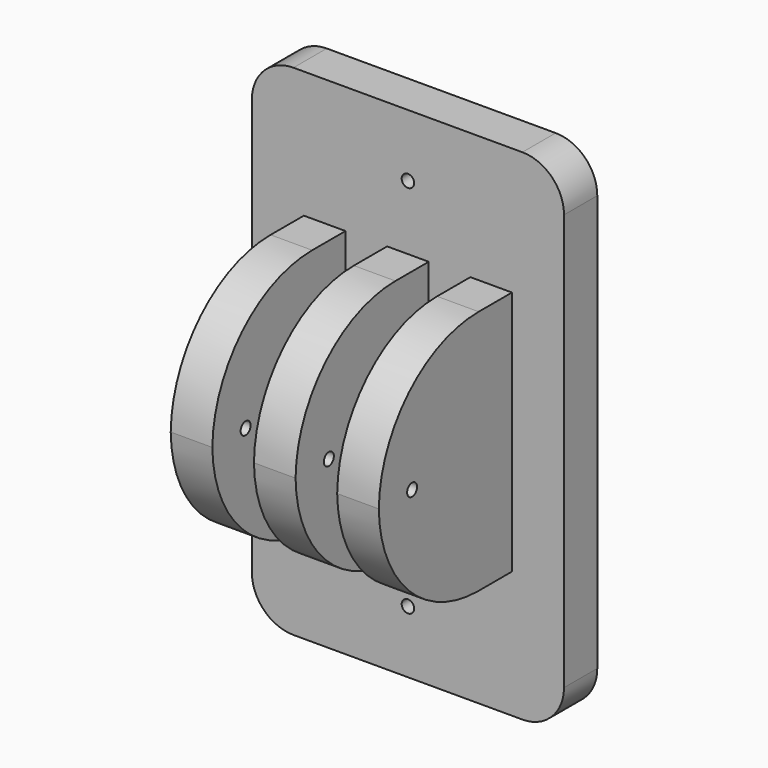
from build123d import *

# Parameters (mm, degrees)
F0_W        = 75
F0_H        = 120
F1_DEPTH    = 10
F2_R        = 1.5
F3_DEPTH    = 41.3
F4_W        = 75
F4_H        = 59.0305535599
F5_DEPTH    = 40
F7_R        = 10
F6_W        = 12.5
F6_H        = 59.0305535599
F6_W_2      = 10
F8_DEPTH    = 40
F9_T1_DEPTH = 160
F9_T3_DEPTH = 160
F9_T5_DEPTH = 160
F10_R       = 1.5
F11_DEPTH   = 57.1


# Not quite as in the source:
# - a fillet or chamfer that OpenCascade refuses, or shapes differently, is made with other operations: its cross-section is extruded or revolved along the edge and cut away or added


with BuildPart() as f1:
    # F0 (on Front) → F1 (new body)
    with BuildSketch(Plane.XZ):
        Rectangle(F0_W, F0_H)
    extrude(amount=F1_DEPTH)

    # F2 (on face) → F3 (cut)
    with BuildSketch(Plane.XZ.offset(10)):
        with Locations((0, -45)):
            Circle(F2_R)
        with Locations((0, 45)):
            Circle(F2_R)
    extrude(amount=-F3_DEPTH, mode=Mode.SUBTRACT)

    # F4 (on face) → F5 (join)
    with BuildSketch(Plane.XZ.offset(10)):
        Rectangle(F4_W, F4_H)
    extrude(amount=F5_DEPTH)

    # F7
    f7_edges = [f1.edges().sort_by_distance(p)[0] for p in [
        (37.5, -5, 60),
        (-37.5, -5, 60),
        (-37.5, -5, -60),
        (37.5, -5, -60),
    ]]
    fillet(f7_edges, radius=F7_R)

    # F6 (on face) → F8 (cut)
    with BuildSketch(Plane.XZ.offset(50)):
        with Locations((-31.25, 0)):
            Rectangle(F6_W, F6_H)
        with Locations((-10, 0)):
            Rectangle(F6_W_2, F6_H)
        with Locations((10, 0)):
            Rectangle(F6_W_2, F6_H)
        with Locations((31.25, 0)):
            Rectangle(F6_W, F6_H)
    extrude(amount=-F8_DEPTH, mode=Mode.SUBTRACT)

    # F9: fillet of radius 30 on 6 edges, made by hand

    # F9_s2 → F9_t1 (cut)
    with BuildSketch(Plane.YZ.offset(-60)):
        with BuildLine():
            ThreePointArc((-50, -0.4847232201), (-41.2132034356, 20.7284802155), (-20, 29.5152767799))
            Line((-20, 29.5152767799), (-50, 29.5152767799))
            Line((-50, 29.5152767799), (-50, -0.4847232201))
        make_face()
        with BuildLine():
            ThreePointArc((-50, 0.4847232201), (-41.2132034356, -20.7284802155), (-20, -29.5152767799))
            Line((-20, -29.5152767799), (-50, -29.5152767799))
            Line((-50, -29.5152767799), (-50, 0.4847232201))
        make_face()
    extrude(amount=F9_T1_DEPTH, mode=Mode.SUBTRACT)

    # F9_s4 → F9_t3 (cut)
    with BuildSketch(Plane.YZ.offset(-80)):
        with BuildLine():
            ThreePointArc((-50, -0.4847232201), (-41.2132034356, 20.7284802155), (-20, 29.5152767799))
            Line((-20, 29.5152767799), (-50, 29.5152767799))
            Line((-50, 29.5152767799), (-50, -0.4847232201))
        make_face()
        with BuildLine():
            ThreePointArc((-50, 0.4847232201), (-41.2132034356, -20.7284802155), (-20, -29.5152767799))
            Line((-20, -29.5152767799), (-50, -29.5152767799))
            Line((-50, -29.5152767799), (-50, 0.4847232201))
        make_face()
    extrude(amount=F9_T3_DEPTH, mode=Mode.SUBTRACT)

    # F9_s6 → F9_t5 (cut)
    with BuildSketch(Plane.YZ.offset(-100)):
        with BuildLine():
            ThreePointArc((-50, -0.4847232201), (-41.2132034356, 20.7284802155), (-20, 29.5152767799))
            Line((-20, 29.5152767799), (-50, 29.5152767799))
            Line((-50, 29.5152767799), (-50, -0.4847232201))
        make_face()
        with BuildLine():
            ThreePointArc((-50, 0.4847232201), (-41.2132034356, -20.7284802155), (-20, -29.5152767799))
            Line((-20, -29.5152767799), (-50, -29.5152767799))
            Line((-50, -29.5152767799), (-50, 0.4847232201))
        make_face()
    extrude(amount=F9_T5_DEPTH, mode=Mode.SUBTRACT)

    # F10 (on face) → F11 (cut)
    with BuildSketch(Plane.YZ.offset(25)):
        with Locations((-39.9960838011, 0)):
            Circle(F10_R)
    extrude(amount=-F11_DEPTH, mode=Mode.SUBTRACT)


solid = f1.part
